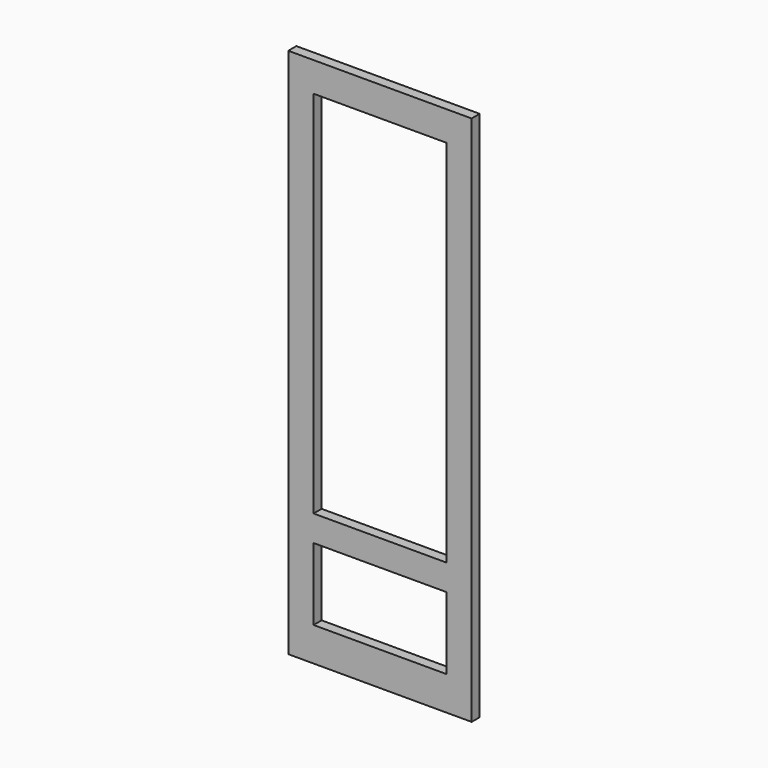
from build123d import *

# Parameters (mm, degrees)
F0_W          = 806.45
F0_H          = 2413
F0_W_2        = 584.2
F0_H_2        = 317.5
F0_H_3        = 1625.6
F1_DEPTH      = 22.225
F1_DEPTH_BACK = 22.225
F2_W          = 1248.5843106929
F2_H          = 271.0993243682
F2_H_2        = 504.0157202398
F3_DEPTH      = 22.226
F3_DEPTH_BACK = 22.226


# Not quite as in the source:
# - a length typed as a fraction of an inch, garbled in the dataset ("3 / 203.2 mm" for 3/8 in), is restored


with BuildPart() as f1:
    # F0 (on Front) → F1 (new body, two sides)
    with BuildSketch(Plane.XZ) as f1_sk:
        Rectangle(F0_W, F0_H)
        with Locations((0, -822.325)):
            Rectangle(F0_W_2, F0_H_2, mode=Mode.SUBTRACT)
        with Locations((0, 263.525)):
            Rectangle(F0_W_2, F0_H_3, mode=Mode.SUBTRACT)
    extrude(amount=F1_DEPTH)
    extrude(f1_sk.sketch, amount=-F1_DEPTH_BACK)

    # F2 (on Front) → F3 (cut, two sides)
    with BuildSketch(Plane.XZ) as f3_sk:
        with Locations((62.8663003445, 1342.0496621841)):
            Rectangle(F2_W, F2_H)
        with Locations((62.8663003445, -1382.3078601199)):
            Rectangle(F2_W, F2_H_2)
    extrude(amount=-F3_DEPTH, mode=Mode.SUBTRACT)
    extrude(f3_sk.sketch, amount=F3_DEPTH_BACK, mode=Mode.SUBTRACT)


solid = f1.part
